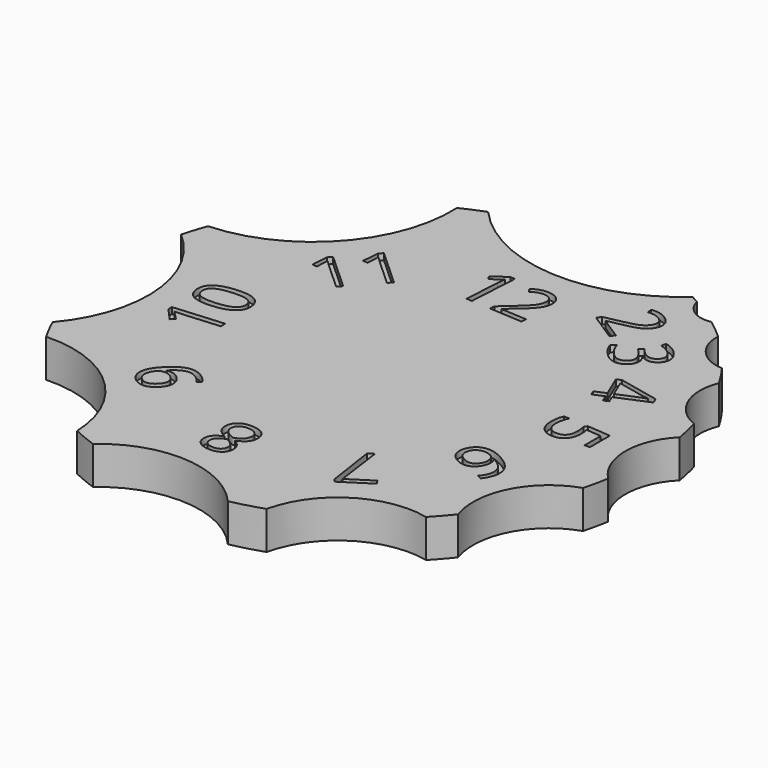
from build123d import *

# Parameters (mm, degrees)
F1_R          = 21
F3_DEPTH      = 3
F4_DEPTH      = 3.001
F5_R          = 9.99999
F6_R          = 8.99999
F7_R          = 7.99999
F8_R          = 6.99999
F9_R          = 5.99999
F10_R         = 4.99999
F11_R         = 3.99999
F12_R         = 2.99999
F13_R         = 1.99999
F14_R         = 10.99999
F15_R         = 11.99999
F16_TEXT_SIZE = 5.5555555556
F17_DEPTH     = 0.5


# Not quite as in the source:
# - a fillet or chamfer is up to 0.001 mm smaller than in the source, because OpenCascade refuses the exact size
# - Text() gives the source's letters only with a copy of the font that has no kerning and outlines rounded to 1/6400 em; it was checked with that copy


with BuildPart() as f3:
    # F1 (on Top) → F3 (new body)
    with BuildSketch(Plane.XY):
        Circle(F1_R)
    extrude(amount=F3_DEPTH)

    # F2 (on Top) → F4 (cut, through all)
    with BuildSketch(Plane.XY):
        Polygon((10.6393431176, 16.3872587233), (12.5955907003, 16.8033060709), (12.1795433527, 18.7595536535), (10.2232957701, 18.343506306), align=None)
        Polygon((13.974139866, 12.5333034268), (16.9697178136, 12.3704760347), (17.1325452058, 15.3660539823), (14.1369672581, 15.5288813745), align=None)
        Polygon((16.5641299889, 6.9941465494), (20.2700273657, 5.4887148398), (21.7754590753, 9.1946122166), (18.0695616985, 10.7000439263), align=None)
        Polygon((17.1647076386, 0), (20.7002415445, -3.5355339059), (24.2357754504, 0), (20.7002415445, 3.5355339059), align=None)
        Polygon((14.5699682527, -7.3620343824), (16.4432877953, -13.0620934953), (22.1433469083, -11.1887739528), (20.2700273657, -5.4887148398), align=None)
        Polygon((8.2934892139, -13.0455303075), (6.7719136852, -19.8781584922), (13.6045418699, -21.3997340209), (15.1261173986, -14.5671058362), align=None)
        Polygon((-0.9988652998, -14.5326072601), (-7.0303003845, -19.7882509713), (-1.7746566732, -25.819686056), (4.2567784114, -20.5640423447), align=None)
        Polygon((-9.2485949334, -10.0372307532), (-18.2410796598, -10.404951362), (-17.8733590509, -19.3974360884), (-8.8808743246, -19.0297154795), align=None)
        Polygon((-26.7596206865, -2.1366632393), (-19.1481772625, -8.6224884763), (-12.6623520256, -1.0110450523), (-20.2737954495, 5.4747801846), align=None)
        Polygon((1.6139958953, 27.6475836597), (-7.3513710381, 19.6712313763), (0.6249812454, 10.7058644429), (9.5903481788, 18.6822167263), align=None)
        Polygon((-20.1772380321, 18.3664797478), (-19.661034663, 7.3785985106), (-8.6731534258, 7.8948018798), (-9.189356795, 18.8826831169), align=None)
    extrude(amount=F4_DEPTH, mode=Mode.SUBTRACT)

    # F5 (radius 10 in the source; OpenCascade refuses exactly that, so slightly less here)
    f5_edges = [f3.edges().sort_by_distance(p)[0] for p in [
        (-12.662352, -1.011045, 1.5),
    ]]
    fillet(f5_edges, radius=F5_R)

    # F6 (radius 9 in the source; OpenCascade refuses exactly that, so slightly less here)
    f6_edges = [f3.edges().sort_by_distance(p)[0] for p in [
        (-9.248595, -10.037231, 1.5),
    ]]
    fillet(f6_edges, radius=F6_R)

    # F7 (radius 8 in the source; OpenCascade refuses exactly that, so slightly less here)
    f7_edges = [f3.edges().sort_by_distance(p)[0] for p in [
        (-0.998865, -14.532607, 1.5),
    ]]
    fillet(f7_edges, radius=F7_R)

    # F8 (radius 7 in the source; OpenCascade refuses exactly that, so slightly less here)
    f8_edges = [f3.edges().sort_by_distance(p)[0] for p in [
        (8.293489, -13.04553, 1.5),
    ]]
    fillet(f8_edges, radius=F8_R)

    # F9 (radius 6 in the source; OpenCascade refuses exactly that, so slightly less here)
    f9_edges = [f3.edges().sort_by_distance(p)[0] for p in [
        (14.569968, -7.362034, 1.5),
    ]]
    fillet(f9_edges, radius=F9_R)

    # F10 (radius 5 in the source; OpenCascade refuses exactly that, so slightly less here)
    f10_edges = [f3.edges().sort_by_distance(p)[0] for p in [
        (17.164708, 0, 1.5),
    ]]
    fillet(f10_edges, radius=F10_R)

    # F11 (radius 4 in the source; OpenCascade refuses exactly that, so slightly less here)
    f11_edges = [f3.edges().sort_by_distance(p)[0] for p in [
        (16.56413, 6.994147, 1.5),
    ]]
    fillet(f11_edges, radius=F11_R)

    # F12 (radius 3 in the source; OpenCascade refuses exactly that, so slightly less here)
    f12_edges = [f3.edges().sort_by_distance(p)[0] for p in [
        (13.97414, 12.533303, 1.5),
    ]]
    fillet(f12_edges, radius=F12_R)

    # F13 (radius 2 in the source; OpenCascade refuses exactly that, so slightly less here)
    f13_edges = [f3.edges().sort_by_distance(p)[0] for p in [
        (10.639343, 16.387259, 1.5),
    ]]
    fillet(f13_edges, radius=F13_R)

    # F14 (radius 11 in the source; OpenCascade refuses exactly that, so slightly less here)
    f14_edges = [f3.edges().sort_by_distance(p)[0] for p in [
        (-8.673153, 7.894802, 1.5),
    ]]
    fillet(f14_edges, radius=F14_R)

    # F15 (radius 12 in the source; OpenCascade refuses exactly that, so slightly less here)
    f15_edges = [f3.edges().sort_by_distance(p)[0] for p in [
        (0.624981, 10.705864, 1.5),
    ]]
    fillet(f15_edges, radius=F15_R)

    # F16 (on face) → F17 (cut)
    with BuildSketch(Plane.XY.offset(3)):
        with Locations(Location((-2.6370263543, 9.8651022991), (0, 0, -3.3409906195))):
            Text('12', F16_TEXT_SIZE, font='Open Sans', text_align=(TextAlign.LEFT, TextAlign.BOTTOM))
        with Locations(Location((-9.4485264207, 4.8983486758), (0, 0, 47.6897400602))):
            Text('11', F16_TEXT_SIZE, font='Open Sans', text_align=(TextAlign.LEFT, TextAlign.BOTTOM))
        with Locations(Location((-10.5542257162, -4.0712772726), (0, 0, 94.565184617))):
            Text('10', F16_TEXT_SIZE, font='Open Sans', text_align=(TextAlign.LEFT, TextAlign.BOTTOM))
        with Locations(Location((-6.5180898187, -9.4636462866), (0, 0, 137.3416339178))):
            Text('9', F16_TEXT_SIZE, font='Open Sans', text_align=(TextAlign.LEFT, TextAlign.BOTTOM))
        with Locations(Location((0.8060783146, -11.9640366118), (0, 0, 176.068090421))):
            Text('8', F16_TEXT_SIZE, font='Open Sans', text_align=(TextAlign.LEFT, TextAlign.BOTTOM))
        with Locations(Location((8.0449552366, -9.5227478072), (0, 0, -147.3084643652))):
            Text('7', F16_TEXT_SIZE, font='Open Sans', text_align=(TextAlign.LEFT, TextAlign.BOTTOM))
        with Locations(Location((12.1693469984, -4.3196107971), (0, 0, -116.8069355545))):
            Text('6', F16_TEXT_SIZE, font='Open Sans', text_align=(TextAlign.LEFT, TextAlign.BOTTOM))
        with Locations(Location((13.2357754504, 1.6085069444), (0, 0, -90))):
            Text('5', F16_TEXT_SIZE, font='Open Sans', text_align=(TextAlign.LEFT, TextAlign.BOTTOM))
        with Locations(Location((11.8968290311, 6.8824877937), (0, 0, -67.108265932))):
            Text('4', F16_TEXT_SIZE, font='Open Sans', text_align=(TextAlign.LEFT, TextAlign.BOTTOM))
        with Locations(Location((9.3606071646, 10.5520630194), (0, 0, -48.1113029746))):
            Text('3', F16_TEXT_SIZE, font='Open Sans', text_align=(TextAlign.LEFT, TextAlign.BOTTOM))
        with Locations(Location((6.4649906756, 12.9315002166), (0, 0, -32.993440429))):
            Text('2', F16_TEXT_SIZE, font='Open Sans', text_align=(TextAlign.LEFT, TextAlign.BOTTOM))
    extrude(amount=-F17_DEPTH, mode=Mode.SUBTRACT)


solid = f3.part
